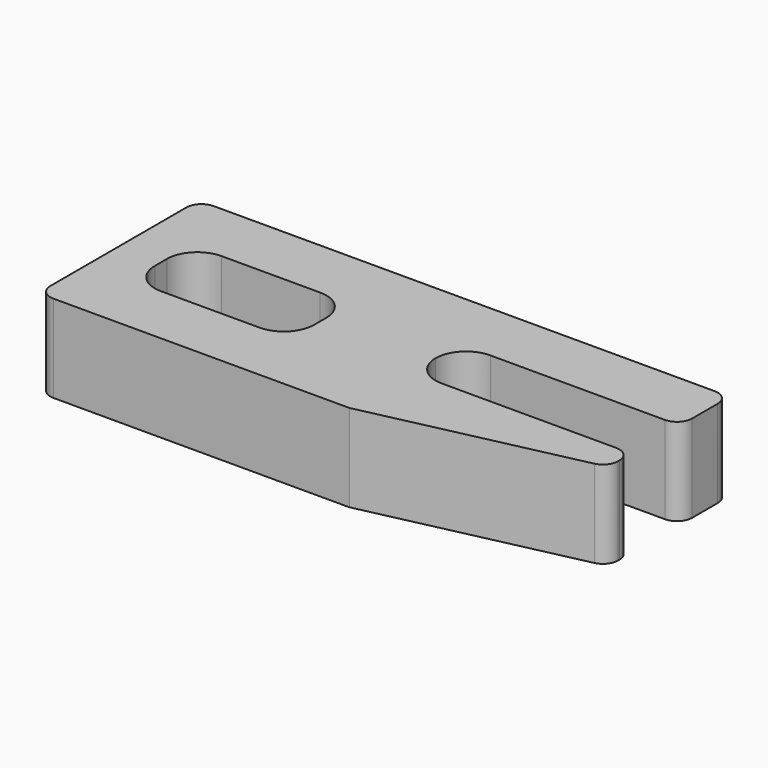
from build123d import *

# Parameters (mm, degrees)
F0_W     = 35
F0_H     = 13.2
F1_DEPTH = 5.76
F2_W     = 10.5
F2_H     = 5
F2_W_2   = 15
F2_H_2   = 4
F3_DEPTH = 25
F4_R     = 1.99999
F5_R     = 1


# Not quite as in the source:
# - a fillet or chamfer is up to 0.001 mm smaller than in the source, because OpenCascade refuses the exact size


with BuildPart() as f1:
    # F0 (on Top) → F1 (new body)
    with BuildSketch(Plane.XY):
        with Locations((-7.6907900348, 3.6986840781)):
            Rectangle(F0_W, F0_H)
    extrude(amount=F1_DEPTH)

    # F2 (on face) → F3 (cut)
    with BuildSketch(Plane.XY.offset(5.76)):
        Polygon((-4.6907900348, -2.9013159219), (9.8092099652, -2.9013159219), (9.8092099652, 0.2986840781), align=None)
        with Locations((-17.1407900348, 3.6986840781)):
            Rectangle(F2_W, F2_H)
        with Locations((2.8092099652, 4.1986840781)):
            Rectangle(F2_W_2, F2_H_2)
    extrude(amount=-F3_DEPTH, mode=Mode.SUBTRACT)

    # F4 (radius 2 in the source; OpenCascade refuses exactly that, so slightly less here)
    f4_edges = [f1.edges().sort_by_distance(p)[0] for p in [
        (-22.39079, 6.198684, 2.88),
        (-11.89079, 6.198684, 2.88),
        (-11.89079, 1.198684, 2.88),
        (-22.39079, 1.198684, 2.88),
        (-4.69079, 2.198684, 2.88),
        (-4.69079, 6.198684, 2.88),
    ]]
    fillet(f4_edges, radius=F4_R)

    # F5
    f5_edges = [f1.edges().sort_by_distance(p)[0] for p in [
        (9.80921, 10.298684, 2.88),
        (9.80921, 6.198684, 2.88),
        (9.80921, 2.198684, 2.88),
        (9.80921, 0.298684, 2.88),
        (-25.19079, -2.901316, 2.88),
        (-25.19079, 10.298684, 2.88),
    ]]
    fillet(f5_edges, radius=F5_R)


solid = f1.part
